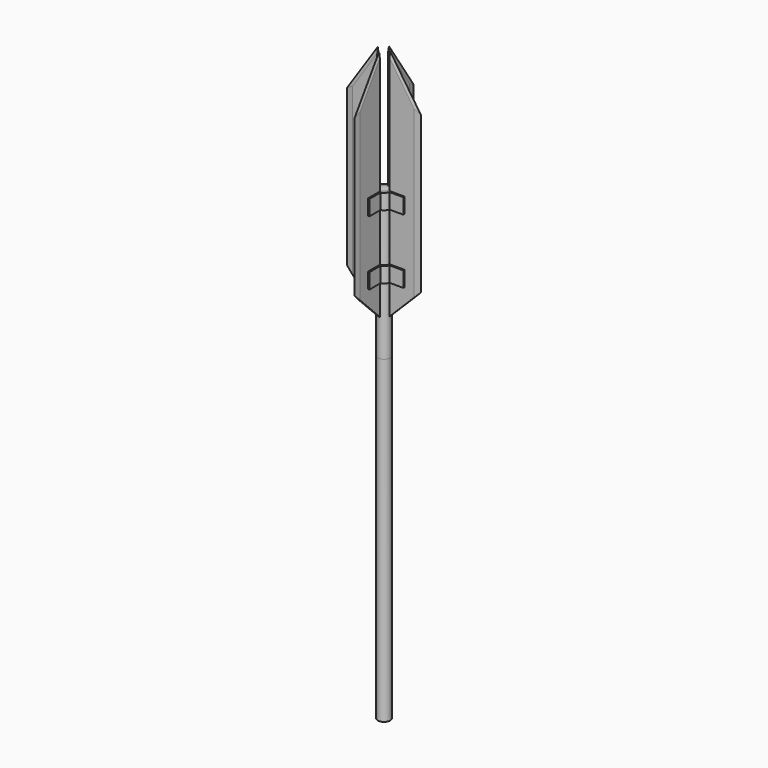
from build123d import *

# Parameters (mm, degrees)
F1_START      = 254
F0_R          = 12.7
F0_R_2        = 9.525
F1_DEPTH      = 660.4
F2_START      = 254
F2_DEPTH      = 965.2
F3_START      = 914.4
F3_DEPTH      = 304.8
F5_DEPTH      = 1.5875
F5_DEPTH_BACK = 1.5875
F7_DEPTH      = 1.5875
F7_DEPTH_BACK = 1.5875
F9_START      = 1054.1
F8_R          = 12.7
F9_DEPTH      = 31.75
F10_START     = 1187.45
F10_DEPTH     = 31.75
F11_SIZE2     = 12.7
F11_SIZE      = 1.5875
F11_2_SIZE2   = 12.7
F11_2_SIZE    = 1.5875
F11_3_SIZE2   = 12.7
F11_3_SIZE    = 1.5875
F11_4_SIZE2   = 12.7
F11_4_SIZE    = 1.5875
F12_SIZE2     = 1.58749
F12_SIZE      = 12.69999
F12_2_SIZE2   = 1.58749
F12_2_SIZE    = 12.69999
F12_3_SIZE2   = 1.58749
F12_3_SIZE    = 12.69999
F12_4_SIZE2   = 1.58749
F12_4_SIZE    = 12.69999
F13_SIZE2     = 1.58749
F13_SIZE      = 6.34999
F13_2_SIZE2   = 1.5875
F13_2_SIZE    = 6.35
F13_3_SIZE2   = 1.58749
F13_3_SIZE    = 6.34999
F13_4_SIZE2   = 1.5875
F13_4_SIZE    = 6.35
F14_SIZE2     = 6.35
F14_SIZE      = 1.5875
F14_2_SIZE2   = 6.34999
F14_2_SIZE    = 1.58749
F14_3_SIZE2   = 6.35
F14_3_SIZE    = 1.5875
F14_4_SIZE2   = 6.34999
F14_4_SIZE    = 1.58749


# Not quite as in the source:
# - a fillet or chamfer is up to 0.001 mm smaller than in the source, because OpenCascade refuses the exact size


with BuildPart() as f1:
    # F0 (on Top) → F1 (new body)
    with BuildSketch(Plane.XY.offset(F1_START)):
        Circle(F0_R)
        Circle(F0_R_2, mode=Mode.SUBTRACT)
    extrude(amount=F1_DEPTH)

    # F0 (on Top) → F2 (join)
    with BuildSketch(Plane.XY.offset(F2_START)):
        Circle(F0_R_2)
    extrude(amount=F2_DEPTH)


with BuildPart() as f3:
    # F0 (on Top) → F3 (new body)
    with BuildSketch(Plane.XY.offset(F3_START)):
        Circle(F0_R)
        Circle(F0_R_2, mode=Mode.SUBTRACT)
    extrude(amount=F3_DEPTH)

    # F4 (on Front) → F5 (join, two sides)
    with BuildSketch(Plane.XZ) as f5_sk:
        Polygon((-12.7, 990.6), (-12.7, 1473.2), (-76.2, 1377.95), (-76.2, 1054.1), align=None)
        Polygon((76.2, 1377.95), (12.7, 1473.2), (12.7, 990.6), (76.2, 1054.1), align=None)
    extrude(amount=F5_DEPTH)
    extrude(f5_sk.sketch, amount=-F5_DEPTH_BACK)

    # F6 (on Right) → F7 (join, two sides)
    with BuildSketch(Plane.YZ) as f7_sk:
        Polygon((-76.2, 1054.1), (-12.7, 990.6), (-12.7, 1473.2), (-76.2, 1377.95), align=None)
        Polygon((12.7, 1473.2), (12.7, 990.6), (76.2, 1054.1), (76.2, 1377.95), align=None)
    extrude(amount=F7_DEPTH)
    extrude(f7_sk.sketch, amount=-F7_DEPTH_BACK)

    # F11
    f11_edges = [f3.edges().sort_by_distance(p)[0] for p in [
        (76.2, -1.5875, 1216.025),
    ]]
    f11_side = f3.faces().sort_by_distance((76.2, 0, 1216.025))[0]
    chamfer(f11_edges, length=F11_SIZE, length2=F11_SIZE2, reference=f11_side)

    # F11#2
    f11_2_edges = [f3.edges().sort_by_distance(p)[0] for p in [
        (1.5875, -76.2, 1216.025),
    ]]
    f11_2_side = f3.faces().sort_by_distance((0, -76.2, 1216.025))[0]
    chamfer(f11_2_edges, length=F11_2_SIZE, length2=F11_2_SIZE2, reference=f11_2_side)

    # F11#3
    f11_3_edges = [f3.edges().sort_by_distance(p)[0] for p in [
        (-76.2, 1.5875, 1216.025),
    ]]
    f11_3_side = f3.faces().sort_by_distance((-76.2, 0, 1216.025))[0]
    chamfer(f11_3_edges, length=F11_3_SIZE, length2=F11_3_SIZE2, reference=f11_3_side)

    # F11#4
    f11_4_edges = [f3.edges().sort_by_distance(p)[0] for p in [
        (-1.5875, 76.2, 1216.025),
    ]]
    f11_4_side = f3.faces().sort_by_distance((0, 76.2, 1216.025))[0]
    chamfer(f11_4_edges, length=F11_4_SIZE, length2=F11_4_SIZE2, reference=f11_4_side)

    # F12 (size 12.7 and 1.5875 in the source; OpenCascade refuses exactly that, so slightly less here)
    f12_edges = [f3.edges().sort_by_distance(p)[0] for p in [
        (-1.5875, -76.2, 1216.025),
    ]]
    f12_side = f3.faces().sort_by_distance((-1.5875, -42.366667, 1224.483333))[0]
    chamfer(f12_edges, length=F12_SIZE, length2=F12_SIZE2, reference=f12_side)

    # F12#2 (size 12.7 and 1.5875 in the source; OpenCascade refuses exactly that, so slightly less here)
    f12_2_edges = [f3.edges().sort_by_distance(p)[0] for p in [
        (-76.2, -1.5875, 1216.025),
    ]]
    f12_2_side = f3.faces().sort_by_distance((-42.366667, -1.5875, 1224.483333))[0]
    chamfer(f12_2_edges, length=F12_2_SIZE, length2=F12_2_SIZE2, reference=f12_2_side)

    # F12#3 (size 12.7 and 1.5875 in the source; OpenCascade refuses exactly that, so slightly less here)
    f12_3_edges = [f3.edges().sort_by_distance(p)[0] for p in [
        (1.5875, 76.2, 1216.025),
    ]]
    f12_3_side = f3.faces().sort_by_distance((1.5875, 42.366667, 1224.483333))[0]
    chamfer(f12_3_edges, length=F12_3_SIZE, length2=F12_3_SIZE2, reference=f12_3_side)

    # F12#4 (size 12.7 and 1.5875 in the source; OpenCascade refuses exactly that, so slightly less here)
    f12_4_edges = [f3.edges().sort_by_distance(p)[0] for p in [
        (76.2, 1.5875, 1216.025),
    ]]
    f12_4_side = f3.faces().sort_by_distance((42.366667, 1.5875, 1224.483333))[0]
    chamfer(f12_4_edges, length=F12_4_SIZE, length2=F12_4_SIZE2, reference=f12_4_side)

    # F13 (size 6.35 and 1.5875 in the source; OpenCascade refuses exactly that, so slightly less here)
    f13_edges = [f3.edges().sort_by_distance(p)[0] for p in [
        (38.100005, 1.5875, 1435.099993),
    ]]
    f13_side = f3.faces().sort_by_distance((36.817176, 1.5875, 1225.870706))[0]
    chamfer(f13_edges, length=F13_SIZE, length2=F13_SIZE2, reference=f13_side)

    # F13#2
    f13_2_edges = [f3.edges().sort_by_distance(p)[0] for p in [
        (-1.5875, 38.1, 1435.1),
    ]]
    f13_2_side = f3.faces().sort_by_distance((-1.5875, 36.817172, 1225.870707))[0]
    chamfer(f13_2_edges, length=F13_2_SIZE, length2=F13_2_SIZE2, reference=f13_2_side)

    # F13#3 (size 6.35 and 1.5875 in the source; OpenCascade refuses exactly that, so slightly less here)
    f13_3_edges = [f3.edges().sort_by_distance(p)[0] for p in [
        (-38.100005, -1.5875, 1435.099993),
    ]]
    f13_3_side = f3.faces().sort_by_distance((-36.817176, -1.5875, 1225.870706))[0]
    chamfer(f13_3_edges, length=F13_3_SIZE, length2=F13_3_SIZE2, reference=f13_3_side)

    # F13#4
    f13_4_edges = [f3.edges().sort_by_distance(p)[0] for p in [
        (1.5875, -38.1, 1435.1),
    ]]
    f13_4_side = f3.faces().sort_by_distance((1.5875, -36.817172, 1225.870707))[0]
    chamfer(f13_4_edges, length=F13_4_SIZE, length2=F13_4_SIZE2, reference=f13_4_side)

    # F14
    f14_edges = [f3.edges().sort_by_distance(p)[0] for p in [
        (38.1, -1.5875, 1435.1),
    ]]
    f14_side = f3.faces().sort_by_distance((41.392614, -0.764347, 1430.161079))[0]
    chamfer(f14_edges, length=F14_SIZE, length2=F14_SIZE2, reference=f14_side)

    # F14#2 (size 1.5875 and 6.35 in the source; OpenCascade refuses exactly that, so slightly less here)
    f14_2_edges = [f3.edges().sort_by_distance(p)[0] for p in [
        (-1.5875, -38.100005, 1435.099993),
    ]]
    f14_2_side = f3.faces().sort_by_distance((-0.764352, -41.392616, 1430.161076))[0]
    chamfer(f14_2_edges, length=F14_2_SIZE, length2=F14_2_SIZE2, reference=f14_2_side)

    # F14#3
    f14_3_edges = [f3.edges().sort_by_distance(p)[0] for p in [
        (-38.1, 1.5875, 1435.1),
    ]]
    f14_3_side = f3.faces().sort_by_distance((-41.392614, 0.764347, 1430.161079))[0]
    chamfer(f14_3_edges, length=F14_3_SIZE, length2=F14_3_SIZE2, reference=f14_3_side)

    # F14#4 (size 1.5875 and 6.35 in the source; OpenCascade refuses exactly that, so slightly less here)
    f14_4_edges = [f3.edges().sort_by_distance(p)[0] for p in [
        (1.5875, 38.100005, 1435.099993),
    ]]
    f14_4_side = f3.faces().sort_by_distance((0.764352, 41.392616, 1430.161076))[0]
    chamfer(f14_4_edges, length=F14_4_SIZE, length2=F14_4_SIZE2, reference=f14_4_side)


with BuildPart() as f9:
    # F8 (on Top) → F9 (new body)
    with BuildSketch(Plane.XY.offset(F9_START)):
        with BuildLine():
            Line((43.7187848225, 4.7625), (15.1437848225, 4.7625))
            ThreePointArc((15.1437848225, 4.7625), (11.2253201513, 11.2253201513), (4.7625, 15.1437848225))
            Line((4.7625, 15.1437848225), (4.7625, 43.7187848225))
            Line((4.7625, 43.7187848225), (-4.7625, 43.7187848225))
            Line((-4.7625, 43.7187848225), (-4.7625, 15.1437848225))
            ThreePointArc((-4.7625, 15.1437848225), (-11.2253201513, 11.2253201513), (-15.1437848225, 4.7625))
            Line((-15.1437848225, 4.7625), (-43.7187848225, 4.7625))
            Line((-43.7187848225, 4.7625), (-43.7187848225, -4.7625))
            Line((-43.7187848225, -4.7625), (-15.1437848225, -4.7625))
            ThreePointArc((-15.1437848225, -4.7625), (-11.2253201513, -11.2253201513), (-4.7625, -15.1437848225))
            Line((-4.7625, -15.1437848225), (-4.7625, -43.7187848225))
            Line((-4.7625, -43.7187848225), (4.7625, -43.7187848225))
            Line((4.7625, -43.7187848225), (4.7625, -15.1437848225))
            ThreePointArc((4.7625, -15.1437848225), (11.2253201513, -11.2253201513), (15.1437848225, -4.7625))
            Line((15.1437848225, -4.7625), (43.7187848225, -4.7625))
            Line((43.7187848225, -4.7625), (43.7187848225, 4.7625))
        make_face()
        Circle(F8_R, mode=Mode.SUBTRACT)
    extrude(amount=F9_DEPTH)


with BuildPart() as f10:
    # F8 (on Top) → F10 (new body)
    with BuildSketch(Plane.XY.offset(F10_START)):
        with BuildLine():
            Line((43.7187848225, 4.7625), (15.1437848225, 4.7625))
            ThreePointArc((15.1437848225, 4.7625), (11.2253201513, 11.2253201513), (4.7625, 15.1437848225))
            Line((4.7625, 15.1437848225), (4.7625, 43.7187848225))
            Line((4.7625, 43.7187848225), (-4.7625, 43.7187848225))
            Line((-4.7625, 43.7187848225), (-4.7625, 15.1437848225))
            ThreePointArc((-4.7625, 15.1437848225), (-11.2253201513, 11.2253201513), (-15.1437848225, 4.7625))
            Line((-15.1437848225, 4.7625), (-43.7187848225, 4.7625))
            Line((-43.7187848225, 4.7625), (-43.7187848225, -4.7625))
            Line((-43.7187848225, -4.7625), (-15.1437848225, -4.7625))
            ThreePointArc((-15.1437848225, -4.7625), (-11.2253201513, -11.2253201513), (-4.7625, -15.1437848225))
            Line((-4.7625, -15.1437848225), (-4.7625, -43.7187848225))
            Line((-4.7625, -43.7187848225), (4.7625, -43.7187848225))
            Line((4.7625, -43.7187848225), (4.7625, -15.1437848225))
            ThreePointArc((4.7625, -15.1437848225), (11.2253201513, -11.2253201513), (15.1437848225, -4.7625))
            Line((15.1437848225, -4.7625), (43.7187848225, -4.7625))
            Line((43.7187848225, -4.7625), (43.7187848225, 4.7625))
        make_face()
        Circle(F8_R, mode=Mode.SUBTRACT)
    extrude(amount=F10_DEPTH)


solid = Compound([f1.part, f3.part, f9.part, f10.part])
